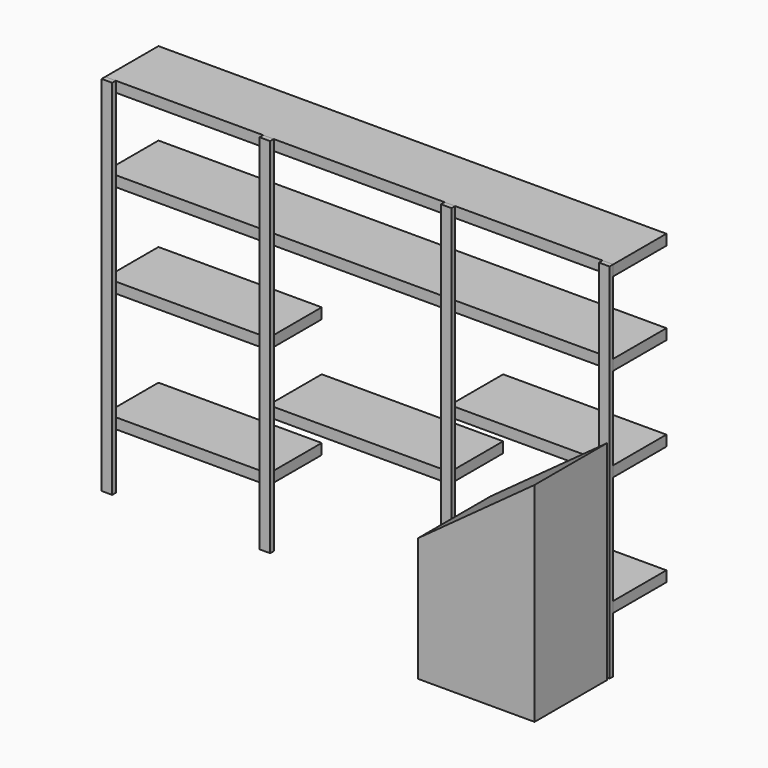
from build123d import *

# Parameters (mm, degrees)
F4_DEPTH = 762
F5_W     = 1524
F5_H     = 88.9
F6_DEPTH = 558.8
F5_W_2   = 1371.6
F5_W_3   = 4267.2
F7_W     = 88.9
F7_H     = 38.1
F8_DEPTH = 3048


with BuildPart() as f4:
    # F3 (on face) → F4 (new body)
    with BuildSketch(Plane(origin=(0, 7912.1, 0), x_dir=(-1, 0, 0), z_dir=(0, 1, 0))):
        Polygon((-3289.3, 1041.4), (-4267.2, 1752.6), (-4267.2, 0), (-3289.3, 0), align=None)
    extrude(amount=-F4_DEPTH)


with BuildPart() as f6:
    # F5 (on face) → F6 (new body)
    with BuildSketch(Plane(origin=(0, 8534.4, 0), x_dir=(-1, 0, 0), z_dir=(0, 1, 0))):
        with Locations((-2133.6, 1022.35)):
            Rectangle(F5_W, F5_H)
    extrude(amount=-F6_DEPTH)


with BuildPart() as f6b:
    # F5 (on face) → F6, piece 2 (new body)
    with BuildSketch(Plane(origin=(0, 8534.4, 0), x_dir=(-1, 0, 0), z_dir=(0, 1, 0))):
        with Locations((-685.8, 1517.65)):
            Rectangle(F5_W_2, F5_H)
    extrude(amount=-F6_DEPTH)


with BuildPart() as f6c:
    # F5 (on face) → F6, piece 3 (new body)
    with BuildSketch(Plane(origin=(0, 8534.4, 0), x_dir=(-1, 0, 0), z_dir=(0, 1, 0))):
        with Locations((-685.8, 514.35)):
            Rectangle(F5_W_2, F5_H)
    extrude(amount=-F6_DEPTH)


with BuildPart() as f6d:
    # F5 (on face) → F6, piece 4 (new body)
    with BuildSketch(Plane(origin=(0, 8534.4, 0), x_dir=(-1, 0, 0), z_dir=(0, 1, 0))):
        with Locations((-2133.6, 3003.55)):
            Rectangle(F5_W_3, F5_H)
    extrude(amount=-F6_DEPTH)


with BuildPart() as f6e:
    # F5 (on face) → F6, piece 5 (new body)
    with BuildSketch(Plane(origin=(0, 8534.4, 0), x_dir=(-1, 0, 0), z_dir=(0, 1, 0))):
        with Locations((-3581.4, 1517.65)):
            Rectangle(F5_W_2, F5_H)
    extrude(amount=-F6_DEPTH)


with BuildPart() as f6f:
    # F5 (on face) → F6, piece 6 (new body)
    with BuildSketch(Plane(origin=(0, 8534.4, 0), x_dir=(-1, 0, 0), z_dir=(0, 1, 0))):
        with Locations((-3581.4, 514.35)):
            Rectangle(F5_W_2, F5_H)
    extrude(amount=-F6_DEPTH)


with BuildPart() as f6g:
    # F5 (on face) → F6, piece 7 (new body)
    with BuildSketch(Plane(origin=(0, 8534.4, 0), x_dir=(-1, 0, 0), z_dir=(0, 1, 0))):
        with Locations((-2133.6, 2305.05)):
            Rectangle(F5_W_3, F5_H)
    extrude(amount=-F6_DEPTH)


with BuildPart() as f8:
    # F7 (on face) → F8 (new body)
    with BuildSketch(Plane.XY):
        with Locations((4222.75, 7956.55)):
            Rectangle(F7_W, F7_H)
    extrude(amount=F8_DEPTH)


with BuildPart() as f8b:
    # F7 (on face) → F8, piece 2 (new body)
    with BuildSketch(Plane.XY):
        with Locations((2895.6, 7956.55)):
            Rectangle(F7_W, F7_H)
    extrude(amount=F8_DEPTH)


with BuildPart() as f8c:
    # F7 (on face) → F8, piece 3 (new body)
    with BuildSketch(Plane.XY):
        with Locations((1371.6, 7956.55)):
            Rectangle(F7_W, F7_H)
    extrude(amount=F8_DEPTH)


with BuildPart() as f8d:
    # F7 (on face) → F8, piece 4 (new body)
    with BuildSketch(Plane.XY):
        with Locations((44.45, 7956.55)):
            Rectangle(F7_W, F7_H)
    extrude(amount=F8_DEPTH)


solid = Compound([f4.part, f6.part, f6b.part, f6c.part, f6d.part, f6e.part, f6f.part, f6g.part, f8.part, f8b.part, f8c.part, f8d.part])
